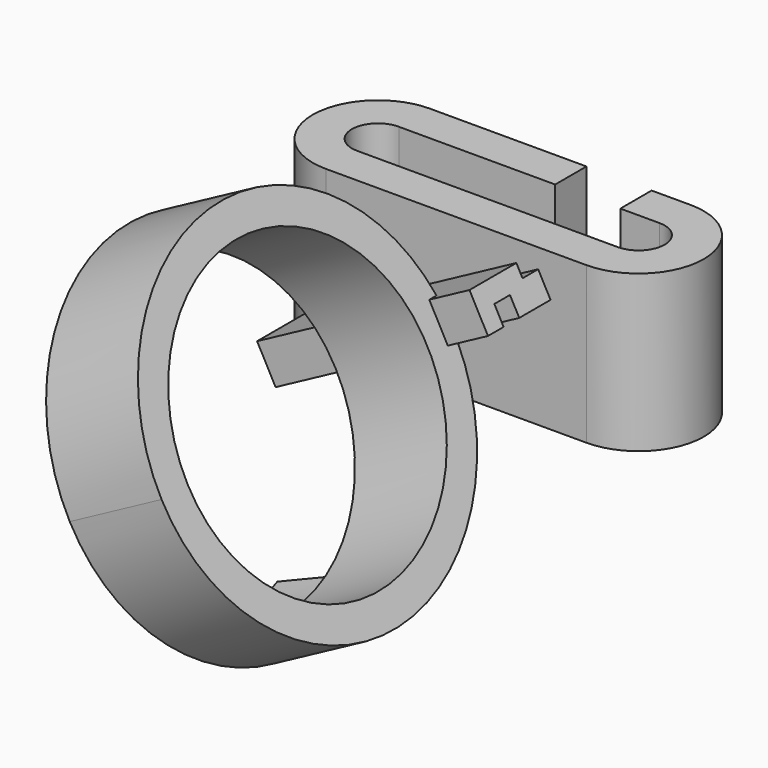
from build123d import *

# Parameters (mm, degrees)
F1_DEPTH       = 12
F5_DEPTH       = 18.5
F7_R           = 11.5
F8_DEPTH       = 8
F11_ANGLE_BACK = 20
F11_ANGLE      = 40


with BuildPart() as f1:
    # F0 (on Top) → F1 (new body)
    with BuildSketch(Plane.XY):
        with BuildLine():
            Line((0, 0), (-20, 0))
            ThreePointArc((-20, 0), (-22, 2), (-20, 4))
            Line((-20, 4), (-8, 4))
            Line((-8, 4), (-8, 7))
            Line((-8, 7), (-20, 7))
            ThreePointArc((-20, 7), (-25, 2), (-20, -3))
            Line((-20, -3), (0, -3))
            ThreePointArc((0, -3), (5, 2), (0, 7))
            Line((0, 7), (-3, 7))
            Line((-3, 7), (-3, 4))
            Line((-3, 4), (0, 4))
            ThreePointArc((0, 4), (2, 2), (0, 0))
        make_face()
    extrude(amount=F1_DEPTH)

    # F4 (on line) → F5 (join)
    with BuildSketch(Plane(origin=(-14.7844431916, 0, -7.9443702008), x_dir=(0, -1, 0), z_dir=(-0.8808807435, 0, -0.4733382677))):
        Polygon((3, 11.0186671228), (3, 9.0186671228), (6, 9.0186671228), (6, 10.5186671228), (7.5, 10.5186671228), (7.5, 9.0186671228), (9, 9.0186671228), (9, 12.0186671228), (4.5, 12.0186671228), (4.5, 11.0186671228), align=None)
    extrude(amount=-F5_DEPTH)

    # F7 (on offset) → F8 (join)
    with BuildSketch(Plane(origin=(-1.5712320387, 0, -0.8442961852), x_dir=(0, -1, 0), z_dir=(-0.8808807435, 0, -0.4733382677))):
        with BuildLine():
            ThreePointArc((36.0992396533, 9.6230288318), (24.609219733, 23.3961911411), (8.9992396533, 14.5616521217))
            Line((8.9992396533, 14.5616521217), (8.9992396533, 4.6844055418))
            ThreePointArc((8.9992396533, 4.6844055418), (24.609219733, -4.1501334776), (36.0992396533, 9.6230288318))
        make_face()
        with Locations((22.0992396533, 9.6230288318)):
            Circle(F7_R, mode=Mode.SUBTRACT)
        with BuildLine():
            Line((8.9992396533, 4.6844055418), (8.9992396533, 14.5616521217))
            ThreePointArc((8.9992396533, 14.5616521217), (8.0992396533, 9.6230288318), (8.9992396533, 4.6844055418))
        make_face()
    extrude(amount=F8_DEPTH)

    # F10 (on offset) → F11 (revolve)
    with BuildSketch(Plane.XZ.offset(21.7), mode=Mode.PRIVATE) as f11_sk:
        Polygon((-6.7922217721, -8.029286104), (-7.7298357056, -6.2843900851), (-11.4623919126, -7.7224527269), align=None)
        Polygon((-21.8758338022, 11.6569236308), (-18.6166158629, 13.9758670161), (-19.5542297964, 15.720763035), align=None)
    revolve(f11_sk.sketch.rotate(Axis((-15.3602525801, -21.7, 2.6705470646), (-0.8808807435, 0, -0.4733382677)), -F11_ANGLE_BACK), axis=Axis((-15.3602525801, -21.7, 2.6705470646), (-0.8808807435, 0, -0.4733382677)), revolution_arc=F11_ANGLE)


solid = f1.part
